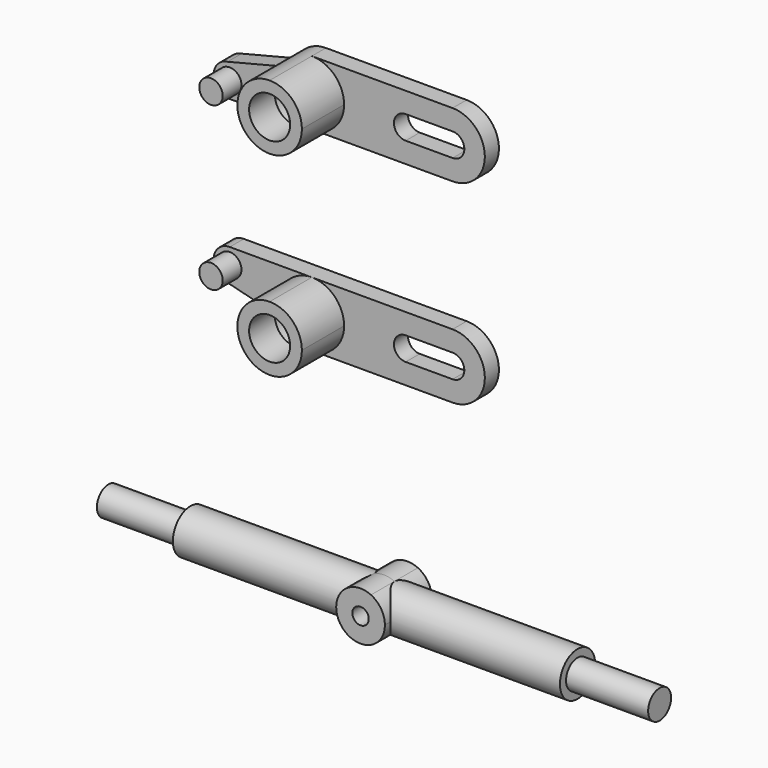
from build123d import *
from build123d import SkipClean  # not in build123d's __all__

# Parameters (mm, degrees)
F0_R     = 4.3
F0_R_2   = 2
F1_DEPTH = 3
F2_DEPTH = 4
F0_R_3   = 3.5
F3_DEPTH = 9
F4_DEPTH = 3.5
F7_DEPTH = 5
F8_DEPTH = 5
F6_W     = 14
F6_H     = 2.45


# Not quite as in the source:
# - after a boolean that leaves OpenCascade's solid faulty, fix() repairs it


with BuildPart() as f1:
    # F0 (on Front) → F1 (new body)
    with BuildSketch(Plane.XZ):
        with BuildLine():
            ThreePointArc((-5.5021138936, 11.1056324095), (-10.1418826672, 13.6522367828), (-10.4850494589, 18.9337975995))
            Line((-10.4850494589, 18.9337975995), (-19.8824234241, 16.5792081218))
            ThreePointArc((-19.8824234241, 16.5792081218), (-17.6970309604, 15.9302831281), (-16.7521138936, 13.8556324095))
            ThreePointArc((-16.7521138936, 13.8556324095), (-17.5575702454, 11.9110887612), (-19.5021138936, 11.1056324095))
            Line((-19.5021138936, 11.1056324095), (-5.5021138936, 11.1056324095))
        make_face()
        with BuildLine():
            ThreePointArc((-0.0021138936, 16.6056324095), (-1.6130265971, 20.494719706), (-5.5021138936, 22.1056324095))
            ThreePointArc((-5.5021138936, 22.1056324095), (-8.4555095203, 21.2454011831), (-10.4850494589, 18.9337975995))
            ThreePointArc((-10.4850494589, 18.9337975995), (-10.1418826672, 13.6522367828), (-5.5021138936, 11.1056324095))
            ThreePointArc((-5.5021138936, 11.1056324095), (-1.6130265971, 12.7165451129), (-0.0021138936, 16.6056324095))
        make_face()
        with Locations((-5.5021138936, 16.6056324095)):
            Circle(F0_R, mode=Mode.SUBTRACT)
        with BuildLine():
            Line((18.4978861064, 22.1056324095), (-5.5021138936, 22.1056324095))
            ThreePointArc((-5.5021138936, 22.1056324095), (-1.6130265971, 20.494719706), (-0.0021138936, 16.6056324095))
            ThreePointArc((-0.0021138936, 16.6056324095), (-1.6130265971, 12.7165451129), (-5.5021138936, 11.1056324095))
            Line((-5.5021138936, 11.1056324095), (18.4978861064, 11.1056324095))
            ThreePointArc((18.4978861064, 11.1056324095), (23.9978861064, 16.6056324095), (18.4978861064, 22.1056324095))
        make_face()
        with BuildLine():
            ThreePointArc((18.4978861064, 18.6056324095), (20.4978861064, 16.6056324095), (18.4978861064, 14.6056324095))
            Line((18.4978861064, 14.6056324095), (10.4978861064, 14.6056324095))
            ThreePointArc((10.4978861064, 14.6056324095), (8.4978861064, 16.6056324095), (10.4978861064, 18.6056324095))
            Line((10.4978861064, 18.6056324095), (18.4978861064, 18.6056324095))
        make_face(mode=Mode.SUBTRACT)
        with BuildLine():
            ThreePointArc((-16.7521138936, 13.8556324095), (-17.6970309604, 15.9302831281), (-19.8824234241, 16.5792081218))
            ThreePointArc((-19.8824234241, 16.5792081218), (-22.245499868, 13.6650192004), (-19.5021138936, 11.1056324095))
            ThreePointArc((-19.5021138936, 11.1056324095), (-17.5575702454, 11.9110887612), (-16.7521138936, 13.8556324095))
        make_face()
        with Locations((-19.5021138936, 13.8556324095)):
            Circle(F0_R_2, mode=Mode.SUBTRACT)
        with Locations((-19.5021138936, 13.8556324095)):
            Circle(F0_R_2)
    extrude(amount=-F1_DEPTH)

    # F0 (on Front) → F2 (join)
    with BuildSketch(Plane.XZ):
        with Locations((-19.5021138936, 13.8556324095)):
            Circle(F0_R_2)
    extrude(amount=F2_DEPTH)

    # F0 (on Front) → F3 (join)
    with BuildSketch(Plane.XZ):
        with BuildLine():
            ThreePointArc((-0.0021138936, 16.6056324095), (-1.6130265971, 20.494719706), (-5.5021138936, 22.1056324095))
            ThreePointArc((-5.5021138936, 22.1056324095), (-8.4555095203, 21.2454011831), (-10.4850494589, 18.9337975995))
            ThreePointArc((-10.4850494589, 18.9337975995), (-10.1418826672, 13.6522367828), (-5.5021138936, 11.1056324095))
            ThreePointArc((-5.5021138936, 11.1056324095), (-1.6130265971, 12.7165451129), (-0.0021138936, 16.6056324095))
        make_face()
        with Locations((-5.5021138936, 16.6056324095)):
            Circle(F0_R, mode=Mode.SUBTRACT)
        with Locations((-5.5021138936, 16.6056324095)):
            Circle(F0_R)
        with Locations((-5.5021138936, 16.6056324095)):
            Circle(F0_R_3, mode=Mode.SUBTRACT)
    with SkipClean():  # cleaning this boolean's faces spoils the solid; the shape is the same uncleaned
        extrude(amount=F3_DEPTH)

    # F4 (cut): a face of the model
    f4_faces = [f1.faces().sort_by_distance(p)[0] for p in [
        (-9.6804915273, 0, 16.6056324095),
    ]]
    extrude(f4_faces, amount=-F4_DEPTH, mode=Mode.SUBTRACT)

    add(f1.part.fix(), mode=Mode.REPLACE)


with BuildPart() as f5_1:
    # F5: instance of F1
    add(f1.part.mirror(Plane.XY), clean=False)


with BuildPart() as f7:
    # F6 (on Front) → F7 (new body)
    with BuildSketch(Plane.XZ):
        with BuildLine():
            Line((8.2020538688, -55.9179931879), (10.9520538688, -55.9179931879))
            ThreePointArc((10.9520538688, -55.9179931879), (10.3091681645, -53.6992887649), (8.5796927522, -52.1679931879))
            ThreePointArc((8.5796927522, -52.1679931879), (6.8020538688, -51.7679931879), (5.0244149853, -52.1679931879))
            ThreePointArc((5.0244149853, -52.1679931879), (3.2949395731, -53.6992887649), (2.6520538688, -55.9179931879))
            Line((2.6520538688, -55.9179931879), (5.4020538688, -55.9179931879))
            ThreePointArc((5.4020538688, -55.9179931879), (6.8020538688, -54.5179931879), (8.2020538688, -55.9179931879))
        make_face()
        with BuildLine():
            ThreePointArc((8.5796927522, -59.6679931879), (10.3091681645, -58.1366976109), (10.9520538688, -55.9179931879))
            Line((10.9520538688, -55.9179931879), (8.2020538688, -55.9179931879))
            ThreePointArc((8.2020538688, -55.9179931879), (6.8020538688, -57.3179931879), (5.4020538688, -55.9179931879))
            Line((5.4020538688, -55.9179931879), (2.6520538688, -55.9179931879))
            ThreePointArc((2.6520538688, -55.9179931879), (3.2949395731, -58.1366976109), (5.0244149853, -59.6679931879))
            ThreePointArc((5.0244149853, -59.6679931879), (6.8020538688, -60.0679931879), (8.5796927522, -59.6679931879))
        make_face()
    extrude(amount=F7_DEPTH)

    # F6 (on Front) → F8 (join)
    with BuildSketch(Plane.XZ):
        with BuildLine():
            Line((8.2020538688, -55.9179931879), (10.9520538688, -55.9179931879))
            ThreePointArc((10.9520538688, -55.9179931879), (10.3091681645, -53.6992887649), (8.5796927522, -52.1679931879))
            ThreePointArc((8.5796927522, -52.1679931879), (6.8020538688, -51.7679931879), (5.0244149853, -52.1679931879))
            ThreePointArc((5.0244149853, -52.1679931879), (3.2949395731, -53.6992887649), (2.6520538688, -55.9179931879))
            Line((2.6520538688, -55.9179931879), (5.4020538688, -55.9179931879))
            ThreePointArc((5.4020538688, -55.9179931879), (6.8020538688, -54.5179931879), (8.2020538688, -55.9179931879))
        make_face()
        with BuildLine():
            ThreePointArc((8.5796927522, -59.6679931879), (10.3091681645, -58.1366976109), (10.9520538688, -55.9179931879))
            Line((10.9520538688, -55.9179931879), (8.2020538688, -55.9179931879))
            ThreePointArc((8.2020538688, -55.9179931879), (6.8020538688, -57.3179931879), (5.4020538688, -55.9179931879))
            Line((5.4020538688, -55.9179931879), (2.6520538688, -55.9179931879))
            ThreePointArc((2.6520538688, -55.9179931879), (3.2949395731, -58.1366976109), (5.0244149853, -59.6679931879))
            ThreePointArc((5.0244149853, -59.6679931879), (6.8020538688, -60.0679931879), (8.5796927522, -59.6679931879))
        make_face()
    extrude(amount=-F8_DEPTH)

    # F6 (on Front) → F9 (revolve)
    with BuildSketch(Plane.XZ):
        with BuildLine():
            ThreePointArc((2.6520538688, -55.9179931879), (3.2949395731, -53.6992887649), (5.0244149853, -52.1679931879))
            Line((5.0244149853, -52.1679931879), (-26.1979461312, -52.1679931879))
            Line((-26.1979461312, -52.1679931879), (-26.1979461312, -53.4679931879))
            Line((-26.1979461312, -53.4679931879), (-26.1979461312, -55.9179931879))
            Line((-26.1979461312, -55.9179931879), (2.6520538688, -55.9179931879))
        make_face()
        with Locations((-33.1979461312, -54.6929931879)):
            Rectangle(F6_W, F6_H)
        with BuildLine():
            ThreePointArc((8.5796927522, -52.1679931879), (10.3091681645, -53.6992887649), (10.9520538688, -55.9179931879))
            Line((10.9520538688, -55.9179931879), (39.8020538688, -55.9179931879))
            Line((39.8020538688, -55.9179931879), (39.8020538688, -53.4679931879))
            Line((39.8020538688, -53.4679931879), (39.8020538688, -52.1679931879))
            Line((39.8020538688, -52.1679931879), (8.5796927522, -52.1679931879))
        make_face()
        with Locations((46.8020538688, -54.6929931879)):
            Rectangle(F6_W, F6_H)
    with SkipClean():  # cleaning this boolean's faces spoils the solid; the shape is the same uncleaned
        revolve(axis=Axis((6.8020538688, 0, -55.9179931879), (1, 0, 0)))


solid = Compound([f1.part, f5_1.part, f7.part])
